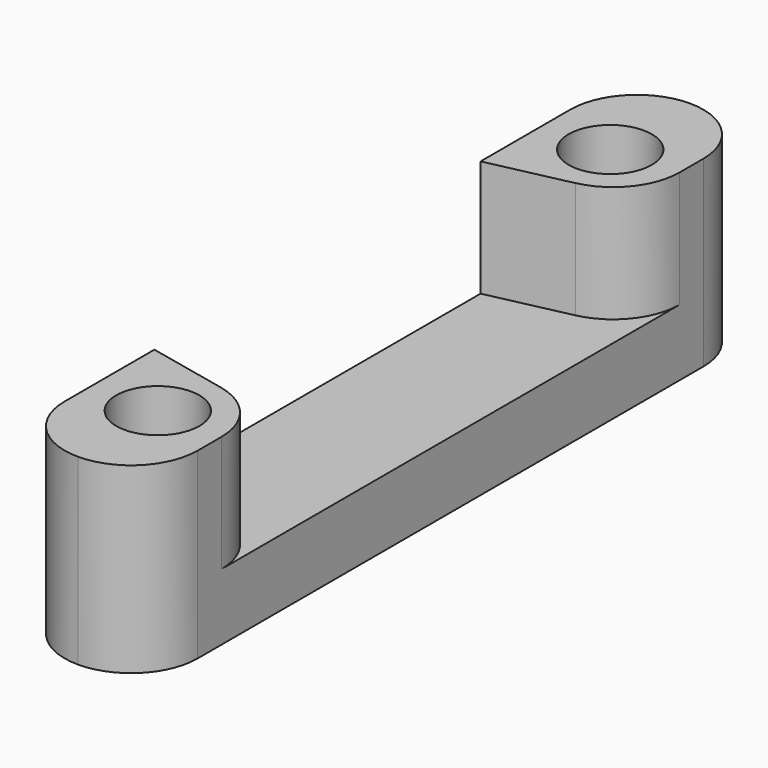
from build123d import *

# Parameters (mm, degrees)
F1_DEPTH = 2
F0_R     = 1.25
F2_DEPTH = 5.5
F3_R     = 1.99999


# Not quite as in the source:
# - a fillet or chamfer is up to 0.001 mm smaller than in the source, because OpenCascade refuses the exact size
# - a feature names something its author has since deleted; it is built from what else it names


with BuildPart() as f1:
    # F0 (on Top) → F1 (new body)
    with BuildSketch(Plane.XY):
        Polygon((-2, 6.1276243068), (-2, -6.1276243068), (2, -7), (2, 7), align=None)
    extrude(amount=F1_DEPTH)

    # F0 (on Top) → F2 (join)
    with BuildSketch(Plane.XY):
        Polygon((-2, 11.5), (-2, 6.1276243068), (2, 7), (2, 11.5), align=None)
        with Locations((0, 8.5)):
            Circle(F0_R, mode=Mode.SUBTRACT)
        Polygon((-2, -11.5), (2, -11.5), (2, -8.2029914483), (2, -7), (-2, -6.1276243068), align=None)
        with Locations((0, -8.5)):
            Circle(F0_R, mode=Mode.SUBTRACT)
    extrude(amount=F2_DEPTH)

    # F3 (radius 2 in the source; OpenCascade refuses exactly that, so slightly less here)
    f3_edges = [f1.edges().sort_by_distance(p)[0] for p in [
        (2, 11.5, 2.75),
        (-2, 11.5, 2.75),
        (2, -11.5, 2.75),
        (-2, -11.5, 2.75),
        (2, -7, 3.75),
        (2, 7, 3.75),
    ]]
    fillet(f3_edges, radius=F3_R)


solid = f1.part
